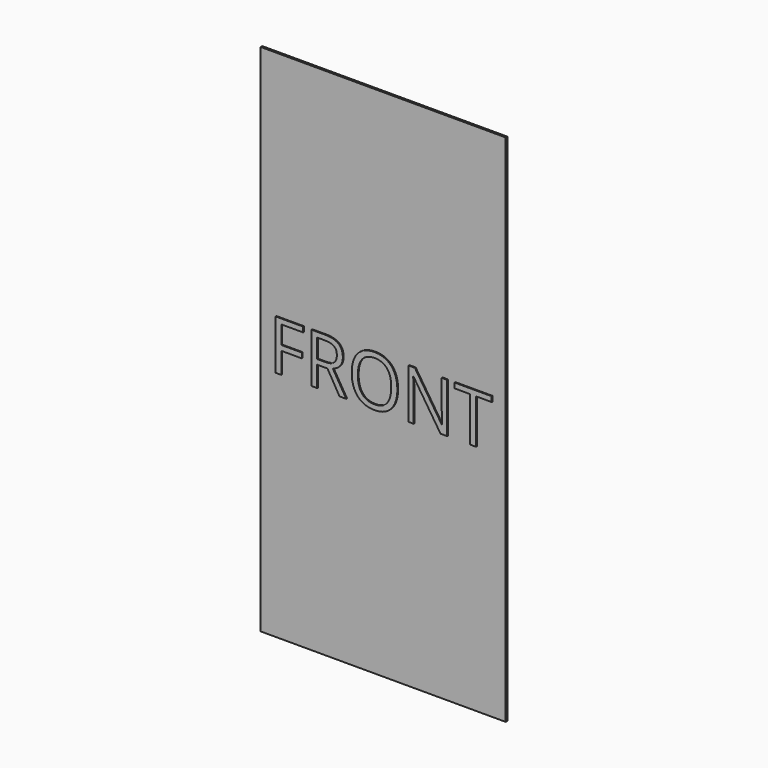
from build123d import *

# Parameters (mm, degrees)
F0_W         = 63.5
F0_H         = 133.35
F1_DEPTH     = 0.254
F2_TEXT_SIZE = 17.9999973625
F3_DEPTH     = 0.254


# Not quite as in the source:
# - Text() gives the source's letters only with a copy of the font that has no kerning and outlines rounded to 1/6400 em; it was checked with that copy


with BuildPart() as f1:
    # F0 (on Front) → F1 (new body, symmetric)
    with BuildSketch(Plane.XZ):
        Rectangle(F0_W, F0_H)
    extrude(amount=F1_DEPTH, both=True)

    # F2 (on face) → F3 (join)
    with BuildSketch(Plane.XZ.offset(0.254)):
        with Locations((-29.4706669138, -6.2366707134)):
            Text('FRONT', F2_TEXT_SIZE, font='Open Sans', text_align=(TextAlign.LEFT, TextAlign.BOTTOM))
    extrude(amount=F3_DEPTH)


solid = f1.part
